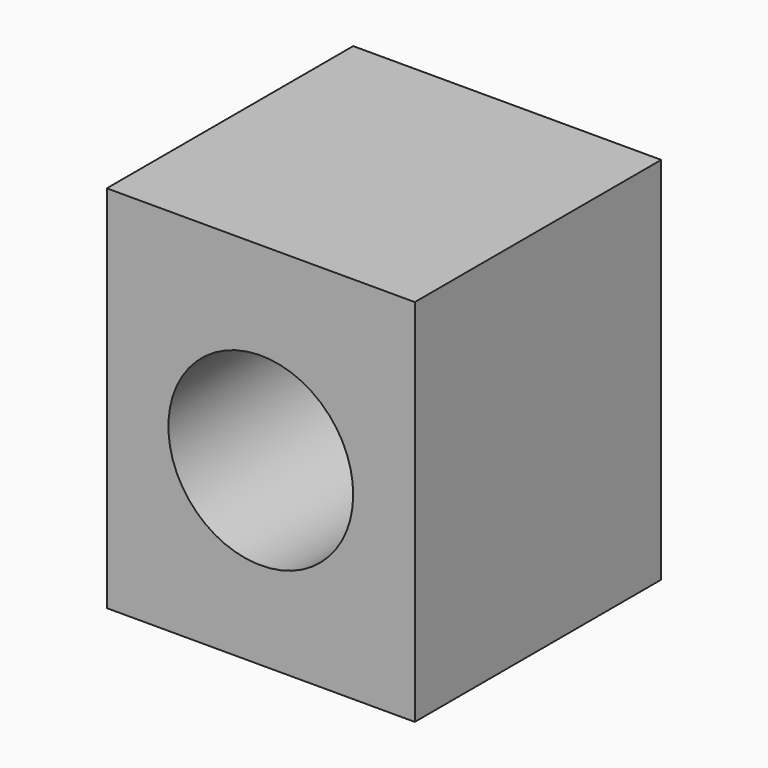
from build123d import *

# Parameters (mm, degrees)
F0_W     = 8
F0_H     = 8
F1_DEPTH = 9.6
F2_R     = 2.4000510118
F3_DEPTH = 25


# Not quite as in the source:
# - the program builds the solid bodies; features that only make, move or delete a surface that nothing else refers to are left out


with BuildPart() as f1:
    # F0 (on Top) → F1 (new body)
    with BuildSketch(Plane.XY):
        Rectangle(F0_W, F0_H)
    extrude(amount=F1_DEPTH)

    # F2 (on face) → F3 (cut)
    with BuildSketch(Plane.XZ.offset(4)):
        with Locations((0, 4.6781064011)):
            Circle(F2_R)
    extrude(amount=-F3_DEPTH, mode=Mode.SUBTRACT)


solid = f1.part
